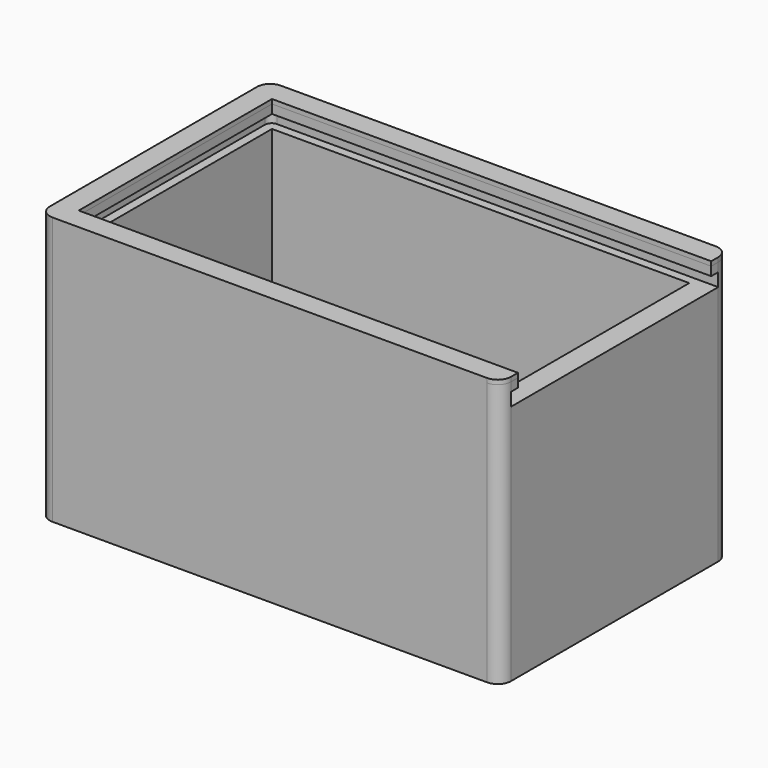
from build123d import *

# Parameters (mm, degrees)
F0_W      = 105
F0_H      = 65
F0_W_2    = 95
F0_H_2    = 55
F1_DEPTH  = 60
F2_DEPTH  = 5
F3_W      = 5
F3_H      = 55
F4_DEPTH  = 5
F6_DEPTH  = 2
F8_DEPTH  = 2
F10_DEPTH = 2
F11_R     = 2.99999
F12_R     = 1.5
F13_DEPTH = 1


# Not quite as in the source:
# - a fillet or chamfer is up to 0.001 mm smaller than in the source, because OpenCascade refuses the exact size


with BuildPart() as f1:
    # F0 (on Top) → F1 (new body)
    with BuildSketch(Plane.XY):
        Rectangle(F0_W, F0_H)
        Rectangle(F0_W_2, F0_H_2, mode=Mode.SUBTRACT)
    extrude(amount=F1_DEPTH)

    # F0 (on Top) → F2 (join)
    with BuildSketch(Plane.XY):
        Rectangle(F0_W_2, F0_H_2)
    extrude(amount=F2_DEPTH)

    # F3 (on face) → F4 (cut)
    with BuildSketch(Plane.XY.offset(60)):
        with Locations((50, 0)):
            Rectangle(F3_W, F3_H)
    extrude(amount=-F4_DEPTH, mode=Mode.SUBTRACT)

    # F5 (on face) → F6 (cut)
    with BuildSketch(Plane.XZ.offset(-27.5)):
        Polygon((47.5, 55), (52.5, 55), (52.5, 58), (-47.5, 58), (-47.5, 55), align=None)
    extrude(amount=-F6_DEPTH, mode=Mode.SUBTRACT)

    # F7 (on face) → F8 (cut)
    with BuildSketch(Plane.YZ.offset(-47.5)):
        Polygon((27.5, 55), (29.5, 55), (29.5, 58), (27.5, 58), (-27.5, 58), (-27.5, 55), align=None)
    extrude(amount=-F8_DEPTH, mode=Mode.SUBTRACT)

    # F9 (on face) → F10 (cut)
    with BuildSketch(Plane(origin=(0, -27.5, 0), x_dir=(-1, 0, 0), z_dir=(0, 1, 0))):
        Polygon((47.5, 55), (49.5, 55), (49.5, 58), (47.5, 58), (-52.5, 58), (-52.5, 55), (-47.5, 55), align=None)
    extrude(amount=-F10_DEPTH, mode=Mode.SUBTRACT)

    # F11 (radius 3 in the source; OpenCascade refuses exactly that, so slightly less here)
    f11_edges = [f1.edges().sort_by_distance(p)[0] for p in [
        (-52.5, -32.5, 30),
        (-52.5, 32.5, 30),
        (52.5, 32.5, 30),
        (52.5, -32.5, 30),
    ]]
    fillet(f11_edges, radius=F11_R)

    # F12
    f12_edges = [f1.edges().sort_by_distance(p)[0] for p in [
        (-49.5, -29.5, 56.5),
        (-49.5, 29.5, 56.5),
    ]]
    fillet(f12_edges, radius=F12_R)

    # F13 (add): a face of the model
    f13_faces = [f1.faces().sort_by_distance(p)[0] for p in [
        (-51.2650910965, 0, 60),
    ]]
    extrude(f13_faces, amount=F13_DEPTH)


solid = f1.part
